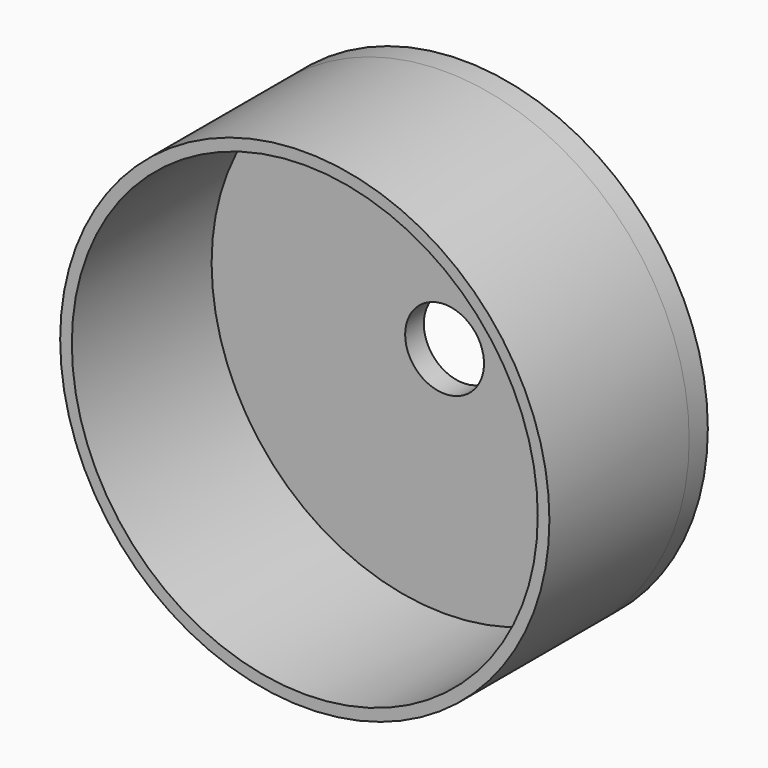
from build123d import *

# Parameters (mm, degrees)
F0_R     = 21
F0_R_2   = 20
F1_DEPTH = 2
F2_R     = 21
F2_R_2   = 20
F3_DEPTH = 15
F4_R     = 3.3845023637
F5_DEPTH = 25


# Not quite as in the source:
# - a feature names something its author has since deleted; it is built from what else it names


with BuildPart() as f1:
    # F0 (on Front) → F1 (new body)
    with BuildSketch(Plane.XZ):
        Circle(F0_R)
        Circle(F0_R_2, mode=Mode.SUBTRACT)
        Circle(F0_R_2)
    extrude(amount=-F1_DEPTH)

    # F2 (on face) → F3 (join)
    with BuildSketch(Plane.XZ):
        Circle(F2_R)
        Circle(F2_R_2, mode=Mode.SUBTRACT)
    extrude(amount=F3_DEPTH)

    # F4 (on face) → F5 (cut)
    with BuildSketch(Plane(origin=(0, 2, 0), x_dir=(-1, 0, 0), z_dir=(0, 1, 0))):
        Circle(F4_R)
    extrude(amount=-F5_DEPTH, mode=Mode.SUBTRACT)


solid = f1.part
